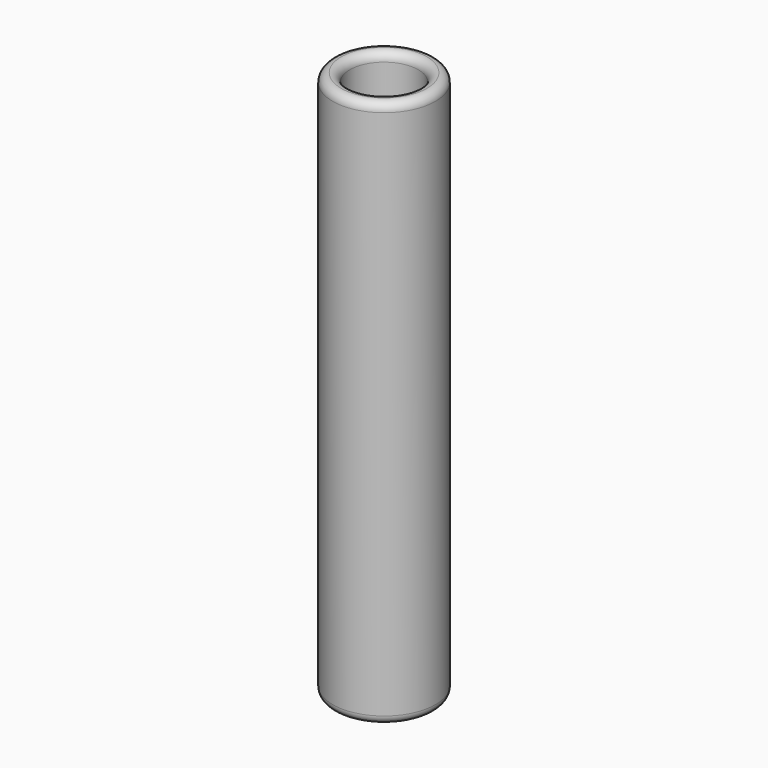
from build123d import *

# Parameters (mm, degrees)
F0_R     = 19.05
F0_R_2   = 12.7
F1_DEPTH = 203.2
F2_R     = 3.17499


# Not quite as in the source:
# - a fillet or chamfer is up to 0.001 mm smaller than in the source, because OpenCascade refuses the exact size


with BuildPart() as f1:
    # F0 (on Top) → F1 (new body)
    with BuildSketch(Plane.XY):
        Circle(F0_R)
        Circle(F0_R_2, mode=Mode.SUBTRACT)
    extrude(amount=F1_DEPTH)

    # F2 (radius 3.175 in the source; OpenCascade refuses exactly that, so slightly less here)
    f2_edges = [f1.edges().sort_by_distance(p)[0] for p in [
        (-12.7, 0, 203.2),
        (-19.05, 0, 203.2),
        (-12.7, 0, 0),
        (-19.05, 0, 0),
    ]]
    fillet(f2_edges, radius=F2_R)


solid = f1.part
